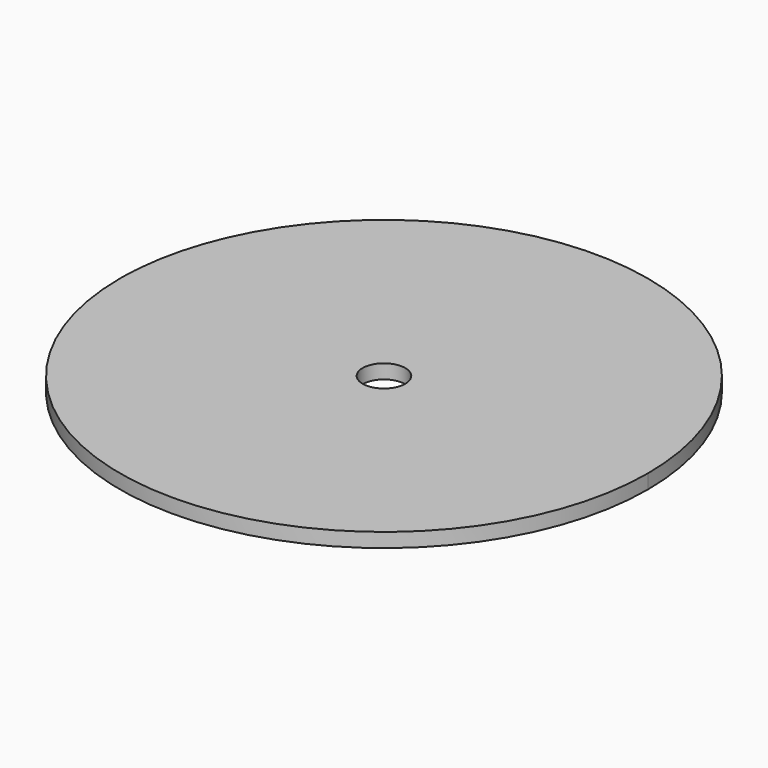
from build123d import *

# Parameters (mm, degrees)
F1_DEPTH = 3.175


# Not quite as in the source:
# - a length typed as a fraction of an inch, garbled in the dataset ("3 / 203.2 mm" for 3/8 in), is restored
# - a feature names something its author has since deleted; it is built from what else it names


with BuildPart() as f1:
    # F0 (on Top) → F1 (new body)
    with BuildSketch(Plane.XY):
        with BuildLine():
            Line((-12.6873488794, 5.5338457858), (-12.6873488794, -31.1003914823))
            ThreePointArc((-12.6873488794, -31.1003914823), (16.4381102813, -21.6348312874), (34.4341148999, 3.1448583573))
            ThreePointArc((34.4341148999, 3.1448583573), (36.2459189148, 10.6981520789), (36.8548431206, 18.4418005177))
            ThreePointArc((36.8548431206, 18.4418005177), (36.6946973558, 22.4220389265), (36.2152954077, 26.3765449929))
            ThreePointArc((36.2152954077, 26.3765449929), (10.5526750719, 26.4063777177), (-12.6873488794, 15.5218814393))
            Line((-12.6873488794, 15.5218814393), (-12.6873488794, 5.5338457858))
        make_face()
        with BuildLine():
            ThreePointArc((34.4341148999, 3.1448583573), (44.4839092315, -60.225850643), (-12.6873488794, -31.1003914823))
            Line((-12.6873488794, -31.1003914823), (-35.5892182517, -31.1003914823))
            ThreePointArc((-35.5892182517, -31.1003914823), (23.3171511206, -90.0067608546), (82.2235204929, -31.1003914823))
            ThreePointArc((82.2235204929, -31.1003914823), (69.3048842905, 5.7111386477), (36.2152954077, 26.3765449929))
            ThreePointArc((36.2152954077, 26.3765449929), (36.6946973558, 22.4220389265), (36.8548431206, 18.4418005177))
            ThreePointArc((36.8548431206, 18.4418005177), (36.2459189148, 10.6981520789), (34.4341148999, 3.1448583573))
        make_face()
        with BuildLine():
            ThreePointArc((34.4341148999, 3.1448583573), (16.4381102813, -21.6348312874), (-12.6873488794, -31.1003914823))
            ThreePointArc((-12.6873488794, -31.1003914823), (44.4839092315, -60.225850643), (34.4341148999, 3.1448583573))
        make_face()
        with BuildLine():
            ThreePointArc((28.0796511206, -31.1003914823), (23.3171511206, -35.8628914823), (18.5546511206, -31.1003914823))
            ThreePointArc((18.5546511206, -31.1003914823), (23.3171511206, -26.3378914823), (28.0796511206, -31.1003914823))
        make_face(mode=Mode.SUBTRACT)
        with BuildLine():
            ThreePointArc((-35.3338578497, -25.6213861535), (-24.3372830845, -29.7111622279), (-12.6873488794, -31.1003914823))
            Line((-12.6873488794, -31.1003914823), (-12.6873488794, 5.5338457858))
            Line((-12.6873488794, 5.5338457858), (-30.6664273508, -7.5263886814))
            ThreePointArc((-30.6664273508, -7.5263886814), (-33.7222633699, -16.3876233128), (-35.3338578497, -25.6213861535))
        make_face()
        with BuildLine():
            Line((-35.5892182517, -31.1003914823), (-12.6873488794, -31.1003914823))
            ThreePointArc((-12.6873488794, -31.1003914823), (-24.3372830845, -29.7111622279), (-35.3338578497, -25.6213861535))
            ThreePointArc((-35.3338578497, -25.6213861535), (-35.5253435202, -28.3579150318), (-35.5892182517, -31.1003914823))
        make_face()
        with BuildLine():
            Line((-30.6664273508, -7.5263886814), (-12.6873488794, 5.5338457858))
            Line((-12.6873488794, 5.5338457858), (-12.6873488794, 15.5218814393))
            ThreePointArc((-12.6873488794, 15.5218814393), (-23.129261611, 5.1306876763), (-30.6664273508, -7.5263886814))
        make_face()
    extrude(amount=F1_DEPTH)


solid = f1.part
